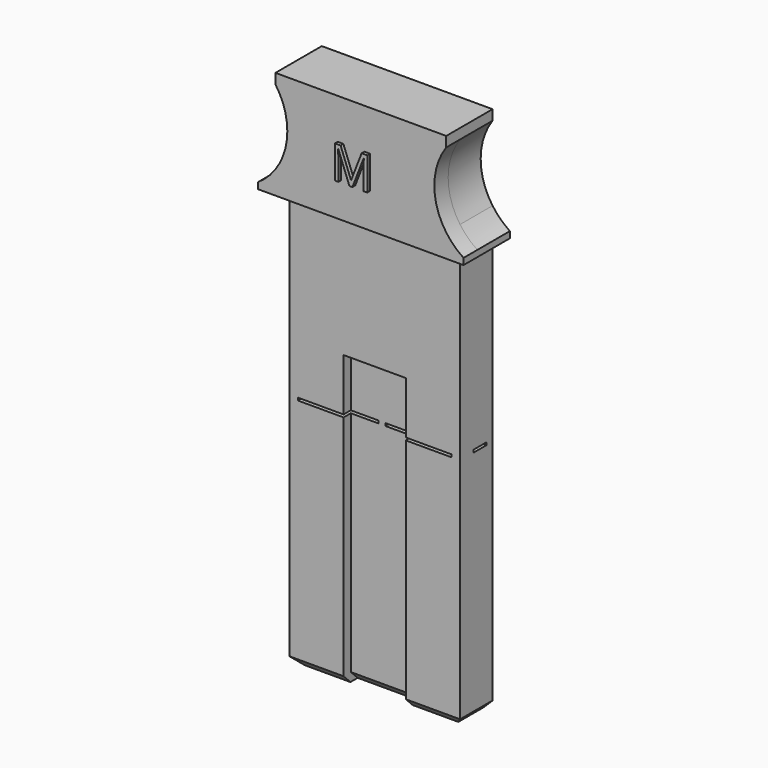
from build123d import *

# Parameters (mm, degrees)
F0_W          = 1
F0_H          = 0.3
F1_DEPTH      = 4.7
F3_DEPTH      = 1.05
F6_DEPTH      = 2
F7_SIZE       = 1
F8_W          = 1.85
F8_H          = 0.3
F9_DEPTH      = 125
F10_TEXT_SIZE = 5.3085904155
F11_DEPTH     = 0.4


# Not quite as in the source:
# - Text() gives the source's letters only with a copy of the font that has no kerning and outlines rounded to 1/6400 em; it was checked with that copy


with BuildPart() as f1:
    # F0 (on Front) → F1 (new body)
    with BuildSketch(Plane.XZ):
        with BuildLine():
            Line((0, 27.35), (0, 0))
            Line((0, 0), (19.75, 0))
            Line((19.75, 0), (19.75, 27.35))
            Line((19.75, 27.35), (18.75, 27.35))
            Line((18.75, 27.35), (10.275, 27.35))
            Line((10.275, 27.35), (10.275, 27.65))
            Line((10.275, 27.65), (18.75, 27.65))
            Line((18.75, 27.65), (19.75, 27.65))
            Line((19.75, 27.65), (19.75, 48.7))
            Line((19.75, 48.7), (19.75, 51.3716775767))
            ThreePointArc((19.75, 51.3716775767), (18.375, 55.7), (19.75, 60.0283224233))
            Line((19.75, 60.0283224233), (19.75, 61.2))
            Line((19.75, 61.2), (0, 61.2))
            Line((0, 61.2), (0, 60.0283224233))
            ThreePointArc((0, 60.0283224233), (1.0229892277, 57.9707377656), (1.375, 55.7))
            ThreePointArc((1.375, 55.7), (1.0229892277, 53.4292622344), (0, 51.3716775767))
            Line((0, 51.3716775767), (0, 48.7))
            Line((0, 48.7), (0, 27.65))
            Line((0, 27.65), (1, 27.65))
            Line((1, 27.65), (9.475, 27.65))
            Line((9.475, 27.65), (9.475, 27.35))
            Line((9.475, 27.35), (1, 27.35))
            Line((1, 27.35), (0, 27.35))
        make_face()
        with BuildLine():
            Line((-2, 48.7), (0, 48.7))
            Line((0, 48.7), (0, 51.3716775767))
            ThreePointArc((0, 51.3716775767), (-0.9094386331, 50.3103878035), (-2, 49.4362650918))
            Line((-2, 49.4362650918), (-2, 48.7))
        make_face()
        with BuildLine():
            Line((19.75, 51.3716775767), (19.75, 48.7))
            Line((19.75, 48.7), (21.75, 48.7))
            Line((21.75, 48.7), (21.75, 49.4362650918))
            ThreePointArc((21.75, 49.4362650918), (20.6594386331, 50.3103878035), (19.75, 51.3716775767))
        make_face()
        with Locations((0.5, 27.5)):
            Rectangle(F0_W, F0_H)
        with Locations((19.25, 27.5)):
            Rectangle(F0_W, F0_H)
    extrude(amount=F1_DEPTH)

    # F2 (on face) → F3 (cut)
    with BuildSketch(Plane.XZ.offset(4.7)):
        Polygon((13.475, 33.7), (6.275, 33.7), (6.275, 2.2), (6.275, 0), (13.475, 0), (13.475, 2.2), align=None)
    extrude(amount=-F3_DEPTH, mode=Mode.SUBTRACT)

    # F5 (on face) → F6 (join)
    with BuildSketch(Plane.XZ.offset(4.7)):
        with BuildLine():
            Line((-2, 48.7), (0, 48.7))
            Line((0, 48.7), (19.75, 48.7))
            Line((19.75, 48.7), (21.75, 48.7))
            Line((21.75, 48.7), (21.75, 49.4362650918))
            ThreePointArc((21.75, 49.4362650918), (18.5052276407, 54.3084342015), (19.75, 60.0283224233))
            Line((19.75, 60.0283224233), (19.75, 61.2))
            Line((19.75, 61.2), (0, 61.2))
            Line((0, 61.2), (0, 60.0283224233))
            ThreePointArc((0, 60.0283224233), (1.2447723593, 54.3084342015), (-2, 49.4362650918))
            Line((-2, 49.4362650918), (-2, 48.7))
        make_face()
    extrude(amount=F6_DEPTH)

    # F7
    f7_edges = [f1.edges().sort_by_distance(p)[0] for p in [
        (0, -2.35, 0),
        (19.75, -2.35, 0),
        (3.1375, -4.7, 0),
        (16.6125, -4.7, 0),
        (9.875, -3.65, 0),
    ]]
    chamfer(f7_edges, length=F7_SIZE)

    # F8 (on face) → F9 (cut, symmetric)
    with BuildSketch(Plane(origin=(9.475, 0, 0), x_dir=(0, -1, 0), z_dir=(-1, 0, 0))):
        with Locations((1.825, 27.5)):
            Rectangle(F8_W, F8_H)
    extrude(amount=F9_DEPTH, both=True, mode=Mode.SUBTRACT)

    # F10 (on face) → F11 (join)
    with BuildSketch(Plane.XZ.offset(6.7)):
        with Locations((6.6712992266, 52.7323260903)):
            Text('M', F10_TEXT_SIZE, font='Open Sans', text_align=(TextAlign.LEFT, TextAlign.BOTTOM))
    extrude(amount=F11_DEPTH)


solid = f1.part
